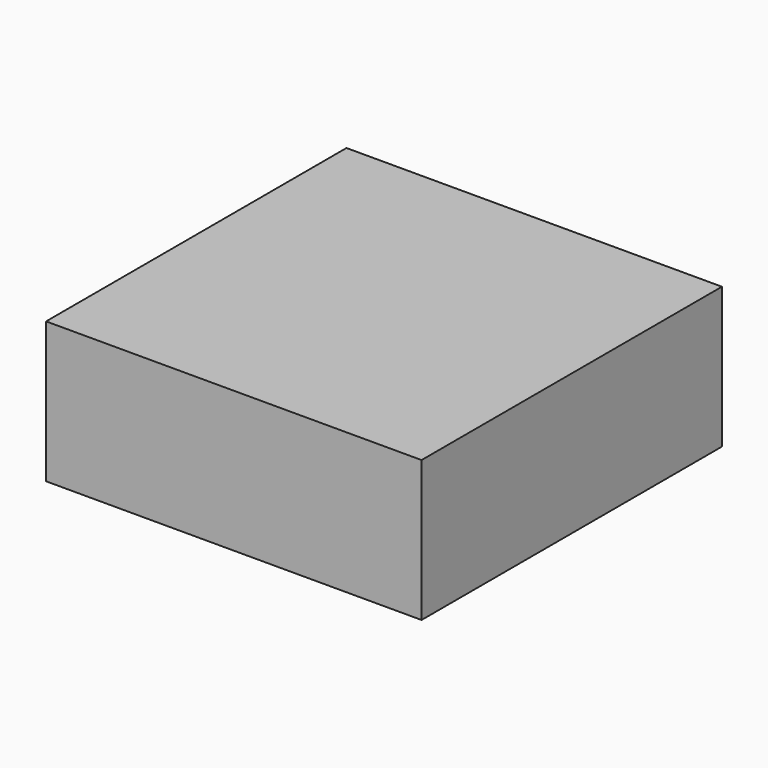
from build123d import *

# Parameters (mm, degrees)
F0_W     = 80
F0_H     = 80
F1_DEPTH = 15


# Not quite as in the source:
# - a feature of the source that left no trace in its solid (it failed there, or was rolled back) is left out


with BuildPart() as f1:
    # F0 (on Top) → F1 (new body, symmetric)
    with BuildSketch(Plane.XY):
        Rectangle(F0_W, F0_H)
    extrude(amount=F1_DEPTH, both=True)


solid = f1.part
